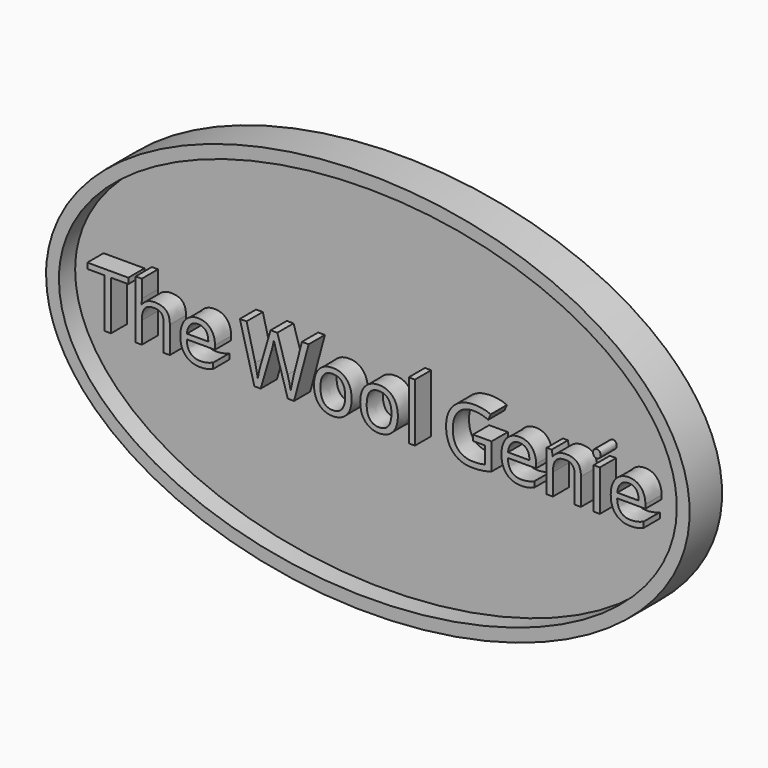
from build123d import *

# Parameters (mm, degrees)
F1_DEPTH     = 4
F3_DEPTH     = 2
F4_TEXT_SIZE = 7.5519967779
F5_DEPTH     = 2


# Not quite as in the source:
# - Text() gives the source's letters only with a copy of the font that has no kerning and outlines rounded to 1/6400 em; it was checked with that copy


with BuildPart() as f1:
    # F0 (on Front) → F1 (new body)
    with BuildSketch(Plane.XZ):
        with BuildLine():
            add(Edge.make_bspline(
                [(-31.75, 0), (-31.75, -32.9955678842), (15.875, -16.4977839421), (63.5, 0), (15.875, 16.4977839421), (-31.75, 32.9955678842), (-31.75, 0)],
                knots=[0, 0, 0, 2.0943951024, 2.0943951024, 4.1887902048, 4.1887902048, 6.2831853072, 6.2831853072, 6.2831853072], degree=2, weights=[1, 0.5, 1, 0.5, 1, 0.5, 1]))
        make_face()
    extrude(amount=F1_DEPTH)

    # F2 (on face) → F3 (cut)
    with BuildSketch(Plane.XZ.offset(4)):
        with BuildLine():
            add(Edge.make_bspline(
                [(-30.48, 0), (-30.48, -30.7958633586), (15.24, -15.3979316793), (60.96, 0), (15.24, 15.3979316793), (-30.48, 30.7958633586), (-30.48, 0)],
                knots=[0, 0, 0, 2.0943951024, 2.0943951024, 4.1887902048, 4.1887902048, 6.2831853072, 6.2831853072, 6.2831853072], degree=2, weights=[1, 0.5, 1, 0.5, 1, 0.5, 1]))
        make_face()
    extrude(amount=-F3_DEPTH, mode=Mode.SUBTRACT)

    # F4 (on face) → F5 (join)
    with BuildSketch(Plane.XZ.offset(2)):
        with Locations((-27.7441835886, -3.0305724672)):
            Text('The Wool Genie', F4_TEXT_SIZE, font='Open Sans', text_align=(TextAlign.LEFT, TextAlign.BOTTOM))
    extrude(amount=F5_DEPTH)


solid = f1.part
